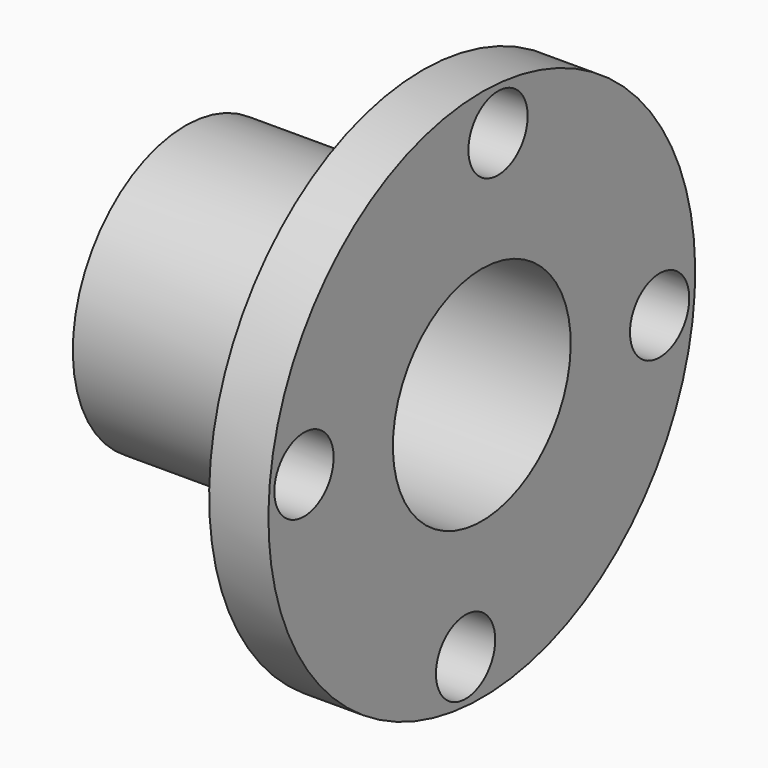
from build123d import *

# Parameters (mm, degrees)
F2_R            = 12.5
F3_DEPTH        = 20.001
F3_COPIES_COUNT = 4


# Not quite as in the source:
# - a pattern or mirror of a feature is missing from the dataset's text; its kind, count and spacing are read off the source's solid


with BuildPart() as f1:
    # F0 (on Front) → F1 (revolve)
    with BuildSketch(Plane.XZ):
        Polygon((-100, 37.5), (0, 37.5), (0, 90), (-20, 90), (-20, 47.5), (-100, 47.5), align=None)
    revolve(axis=Axis((-167.8846976696, 0, 0), (-1, 0, 0)))

    # F2 (on face) → F3 (cut, through all)
    with BuildSketch(Plane(origin=(-20, 0, 0), x_dir=(0, -1, 0), z_dir=(-1, 0, 0))):
        with Locations((-6.848233752, 75)):
            Circle(F2_R)
    f3 = extrude(amount=-F3_DEPTH, mode=Mode.SUBTRACT)

    # F3_copies: F3 ×4 about axis
    f3_copies_axis = Axis((0, 0, 0), (1, 0, 0))
    for i in range(1, F3_COPIES_COUNT):
        add(f3.rotate(f3_copies_axis, i * 360 / F3_COPIES_COUNT), mode=Mode.SUBTRACT)


solid = f1.part
